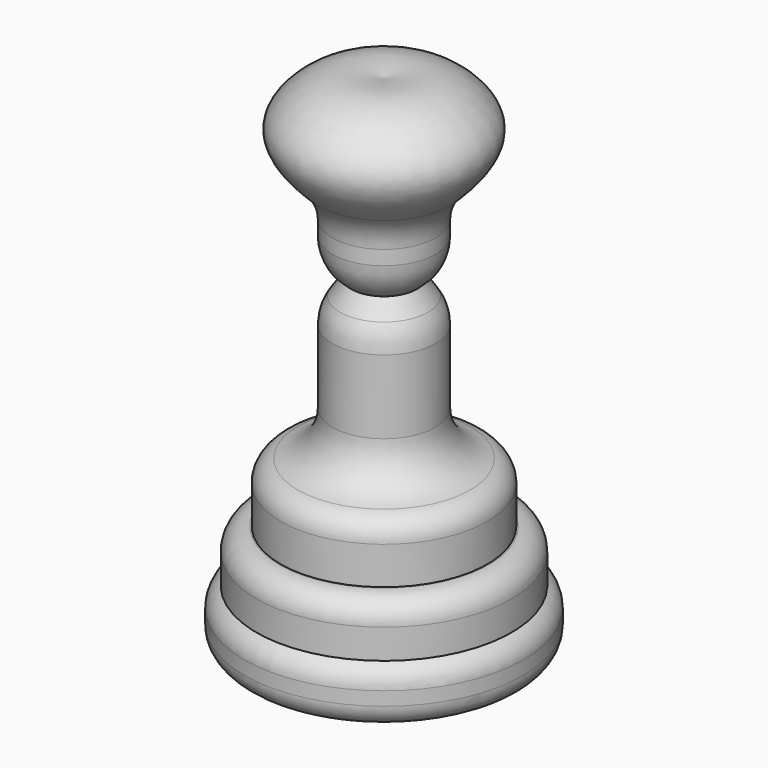
from build123d import *


# Not quite as in the source:
# - a fillet or chamfer that OpenCascade refuses, or shapes differently, is made with other operations: its cross-section is extruded or revolved along the edge and cut away or added


with BuildPart() as f1:
    # F0 (on Front) → F1 (revolve)
    with BuildSketch(Plane.XZ):
        Polygon((-15.6518872827, -56.4240813255), (0, -56.4240813255), (0, -50.1076057553), (-14.2983561382, -50.1076057553), (-15.6518872827, -50.1076057553), align=None)
        Polygon((-14.2983561382, -50.1076057553), (0, -50.1076057553), (0, -44.2423075438), (-11.5912947804, -44.2423075438), (-14.2983561382, -44.2423075438), align=None)
        Polygon((-11.5912947804, -44.2423075438), (0, -44.2423075438), (0, -37.4746546149), (-5.7956473902, -37.4746546149), (-11.5912947804, -37.4746546149), align=None)
        with BuildLine():
            Line((-5.7956473902, -37.4746546149), (0, -37.4746546149))
            Line((0, -37.4746546149), (0, -11.7575740442))
            add(Edge.make_bspline(
                [(-5.7956473902, -11.7575740442), (-3.8637649268, -11.7575740442), (-1.9318824634, -11.7575740442), (0, -11.7575740442)],
                knots=[0, 0, 0, 0, 5.7956473902, 5.7956473902, 5.7956473902, 5.7956473902], degree=3))
            Line((-5.7956473902, -11.7575740442), (-5.7956473902, -18.2568924401))
            Line((-5.7956473902, -18.2568924401), (-3.6957010161, -19.6531694382))
            Line((-3.6957010161, -19.6531694382), (-5.7956473902, -22.8114072233))
            Line((-5.7956473902, -22.8114072233), (-5.7956473902, -37.4746546149))
        make_face()
        with BuildLine():
            add(Edge.make_bspline(
                [(-5.7956473902, -11.7575740442), (-3.8637649268, -11.7575740442), (-1.9318824634, -11.7575740442), (0, -11.7575740442)],
                knots=[0, 0, 0, 0, 5.7956473902, 5.7956473902, 5.7956473902, 5.7956473902], degree=3))
            Line((0, -11.7575740442), (0, 0))
            add(Edge.make_bspline(
                [(-5.7956473902, -11.7575740442), (-7.4873116025, -10.1638177583), (-10.4160184448, -7.4046147761), (-10.9671540458, -3.3330390808), (-5.8286728705, 0.9272611073), (-1.9459726357, 0.3095772882), (0, 0)],
                knots=[0, 0, 0, 0, 0.2748295004, 0.475800713, 0.7372762752, 1, 1, 1, 1], degree=3))
        make_face()
    revolve(axis=Axis((0, 0, -28.2120406628), (0, 0, -1)))

    # F2: fillet of radius 2.54 on 5 edges, made by hand

    # F2_s1 → F2_t2 (revolve, cut)
    with BuildSketch(Plane.XZ):
        with BuildLine():
            ThreePointArc((-9.0512947804, -37.4746546149), (-10.8473460046, -38.2186033907), (-11.5912947804, -40.0146546149))
            Line((-11.5912947804, -40.0146546149), (-11.5912947804, -37.4746546149))
            Line((-11.5912947804, -37.4746546149), (-9.0512947804, -37.4746546149))
        make_face()
    revolve(axis=Axis((0, 0, -37.4746546149), (0, 0, -1)), mode=Mode.SUBTRACT)

    # F2_s3 → F2_t4 (revolve, cut)
    with BuildSketch(Plane.XZ):
        with BuildLine():
            ThreePointArc((-14.2983561382, -50.1076057553), (-15.2873448085, -51.0423662482), (-15.6518872827, -52.3534667606))
            Line((-15.6518872827, -52.3534667606), (-15.6518872827, -50.1076057553))
            Line((-15.6518872827, -50.1076057553), (-14.2983561382, -50.1076057553))
        make_face()
    revolve(axis=Axis((0, 0, -50.1076057553), (0, 0, -1)), mode=Mode.SUBTRACT)

    # F2_s5 → F2_t6 (revolve, cut)
    with BuildSketch(Plane.XZ):
        with BuildLine():
            ThreePointArc((-13.1118872827, -56.4240813255), (-14.9079385069, -55.6801325497), (-15.6518872827, -53.8840813255))
            Line((-15.6518872827, -53.8840813255), (-15.6518872827, -56.4240813255))
            Line((-15.6518872827, -56.4240813255), (-13.1118872827, -56.4240813255))
        make_face()
    revolve(axis=Axis((0, 0, -56.4240813255), (0, 0, -1)), mode=Mode.SUBTRACT)

    # F2_s7 → F2_t8 (revolve, cut)
    with BuildSketch(Plane.XZ):
        with BuildLine():
            ThreePointArc((-11.7583561382, -44.2423075438), (-13.5544073624, -44.9862563195), (-14.2983561382, -46.7823075438))
            Line((-14.2983561382, -46.7823075438), (-14.2983561382, -44.2423075438))
            Line((-14.2983561382, -44.2423075438), (-11.7583561382, -44.2423075438))
        make_face()
    revolve(axis=Axis((0, 0, -44.2423075438), (0, 0, -1)), mode=Mode.SUBTRACT)

    # F3: fillet of radius 5.08 on 6 edges, made by hand

    # F3_s1 → F3_t2 (revolve)
    with BuildSketch(Plane.XZ):
        with BuildLine():
            ThreePointArc((-9.659412317, -37.5485254493), (-6.8765928662, -35.7489916373), (-5.7956473902, -32.616267118))
            Line((-5.7956473902, -32.616267118), (-5.2876473902, -32.616267118))
            Line((-5.2876473902, -32.616267118), (-5.2876473902, -37.4746546149))
            Line((-5.2876473902, -37.4746546149), (-5.7956473902, -37.9826546149))
            ThreePointArc((-5.7956473902, -37.9826546149), (-9.0512947804, -37.9826546149), (-9.5377888097, -38.0417512824))
            Line((-9.5377888097, -38.0417512824), (-9.659412317, -37.5485254493))
        make_face()
    revolve(axis=Axis((0, 0, -37.4746546149), (0, 0, -1)))

    # F3_s3 → F3_t4 (revolve)
    with BuildSketch(Plane.XZ):
        with BuildLine():
            ThreePointArc((-5.7956473902, -13.9279319037), (-6.1893860399, -11.9669743425), (-7.3095665071, -10.309995042))
            Line((-7.3095665071, -10.309995042), (-7.2382448894, -10.2376363048))
            ThreePointArc((-7.2382448894, -10.2376363048), (-6.4865657886, -10.9644490522), (-5.7259772163, -11.6836238794))
            Line((-5.7259772163, -11.6836238794), (-5.6940473902, -11.7575740442))
            Line((-5.6940473902, -11.7575740442), (-5.6940473902, -13.9279319037))
            Line((-5.6940473902, -13.9279319037), (-5.7956473902, -13.9279319037))
        make_face()
    revolve(axis=Axis((0, 0, -11.7575740442), (0, 0, -1)))

    # F3_s5 → F3_t6 (revolve, cut)
    with BuildSketch(Plane.XZ):
        with BuildLine():
            ThreePointArc((-5.7956473902, -24.3461346524), (-5.5785694611, -22.8769890052), (-4.945887968, -21.5334020568))
            Line((-4.945887968, -21.5334020568), (-5.0304927795, -21.4771474049))
            Line((-5.0304927795, -21.4771474049), (-5.8972473902, -22.7807126748))
            Line((-5.8972473902, -22.7807126748), (-5.8972473902, -24.3461346524))
            Line((-5.8972473902, -24.3461346524), (-5.7956473902, -24.3461346524))
        make_face()
    revolve(axis=Axis((0, 0, -22.8114072233), (0, 0, -1)), mode=Mode.SUBTRACT)

    # F3_s7 → F3_t8 (revolve, cut)
    with BuildSketch(Plane.XZ):
        with BuildLine():
            ThreePointArc((-3.6957010161, -19.6531694382), (-5.2403060745, -17.8486021825), (-5.7956473902, -15.5390862613))
            Line((-5.7956473902, -15.5390862613), (-5.8972473902, -15.5390862613))
            Line((-5.8972473902, -15.5390862613), (-5.8972473902, -18.2568924401))
            Line((-5.8972473902, -18.2568924401), (-5.8519020421, -18.3414972517))
            ThreePointArc((-5.8519020421, -18.3414972517), (-4.8019288551, -19.0396357507), (-3.7553020886, -19.7354511018))
            Line((-3.7553020886, -19.7354511018), (-3.6957010161, -19.6531694382))
        make_face()
    revolve(axis=Axis((0, 0, -18.2568924401), (0, 0, -1)), mode=Mode.SUBTRACT)


solid = f1.part
